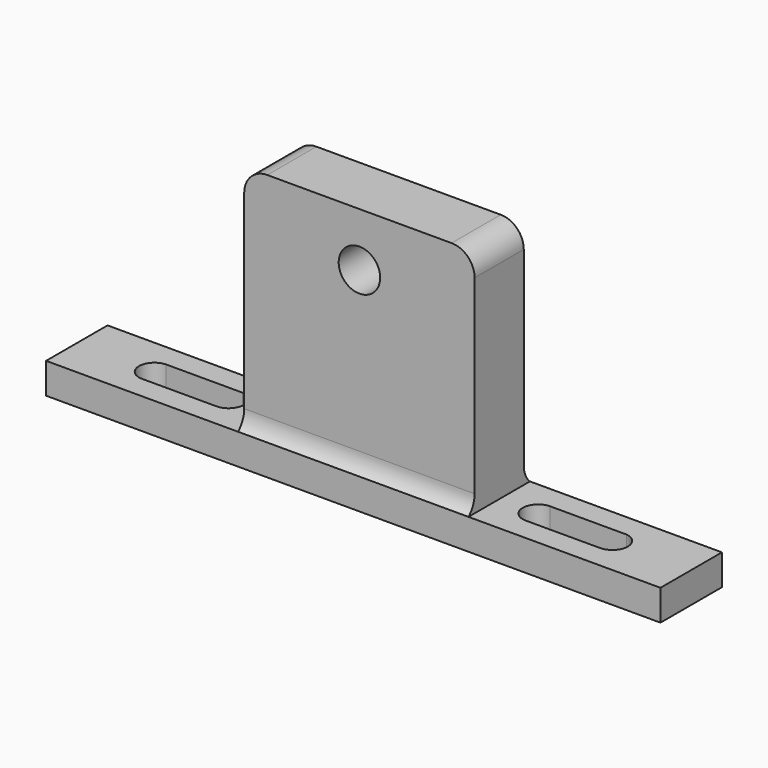
from build123d import *

# Parameters (mm, degrees)
F0_W        = 80
F0_H        = 10
F2_DEPTH    = 4
F1_W        = 30
F1_H        = 34
F1_R        = 2.7
F3_DEPTH    = 4
F4_T1_DEPTH = 30
F4_T3_DEPTH = 30
F4_T5_DEPTH = 23
F4_T7_DEPTH = 23


# Not quite as in the source:
# - a fillet or chamfer that OpenCascade refuses, or shapes differently, is made with other operations: its cross-section is extruded or revolved along the edge and cut away or added


with BuildPart() as f2:
    # F0 (on Top) → F2 (new body)
    with BuildSketch(Plane.XY):
        Rectangle(F0_W, F0_H)
        with BuildLine():
            ThreePointArc((-29.8963663541, -2.000000095), (-31.8970374873, -0.0504918144), (-30, 1.999999905))
            Line((-30, 1.999999905), (-20, 1.999999905))
            ThreePointArc((-20, 1.999999905), (-18.2234549617, -0.1070915702), (-20.226663407, -2.000000095))
            Line((-20.226663407, -2.000000095), (-29.8963663541, -2.000000095))
        make_face(mode=Mode.SUBTRACT)
        with BuildLine():
            ThreePointArc((20.0609671511, -2.000000095), (18.0607348524, -0.030022587), (20, 1.999999905))
            Line((20, 1.999999905), (30, 1.999999905))
            ThreePointArc((30, 1.999999905), (31.7352004336, -0.1259018267), (29.7306719608, -2.000000095))
            Line((29.7306719608, -2.000000095), (20.0609671511, -2.000000095))
        make_face(mode=Mode.SUBTRACT)
    extrude(amount=F2_DEPTH)

    # F1 (on Front) → F3 (join, symmetric)
    with BuildSketch(Plane.XZ):
        with Locations((0, 17)):
            Rectangle(F1_W, F1_H)
        with Locations((0, 27)):
            Circle(F1_R, mode=Mode.SUBTRACT)
    extrude(amount=F3_DEPTH, both=True)

    # F4: fillet of radius 3 on 4 edges, made by hand

    # F4_s2 → F4_t1 (join)
    with BuildSketch(Plane.YZ.offset(-15)):
        with BuildLine():
            ThreePointArc((5, 4), (4.2613872125, 5.0113231061), (4, 6.2360679775))
            Line((4, 6.2360679775), (4, 4))
            Line((4, 4), (5, 4))
        make_face()
    extrude(amount=F4_T1_DEPTH)

    # F4_s4 → F4_t3 (join)
    with BuildSketch(Plane.YZ.offset(-15)):
        with BuildLine():
            ThreePointArc((-4, 6.2360679775), (-4.2613872125, 5.0113231061), (-5, 4))
            Line((-5, 4), (-4, 4))
            Line((-4, 4), (-4, 6.2360679775))
        make_face()
    extrude(amount=F4_T3_DEPTH)

    # F4_s6 → F4_t5 (cut)
    with BuildSketch(Plane.XZ.offset(-11.5)):
        with BuildLine():
            ThreePointArc((15, 31), (14.1213203436, 33.1213203436), (12, 34))
            Line((12, 34), (15, 34))
            Line((15, 34), (15, 31))
        make_face()
    extrude(amount=F4_T5_DEPTH, mode=Mode.SUBTRACT)

    # F4_s8 → F4_t7 (cut)
    with BuildSketch(Plane.XZ.offset(-11.5)):
        with BuildLine():
            ThreePointArc((-15, 31), (-14.1213203436, 33.1213203436), (-12, 34))
            Line((-12, 34), (-15, 34))
            Line((-15, 34), (-15, 31))
        make_face()
    extrude(amount=F4_T7_DEPTH, mode=Mode.SUBTRACT)


solid = f2.part
